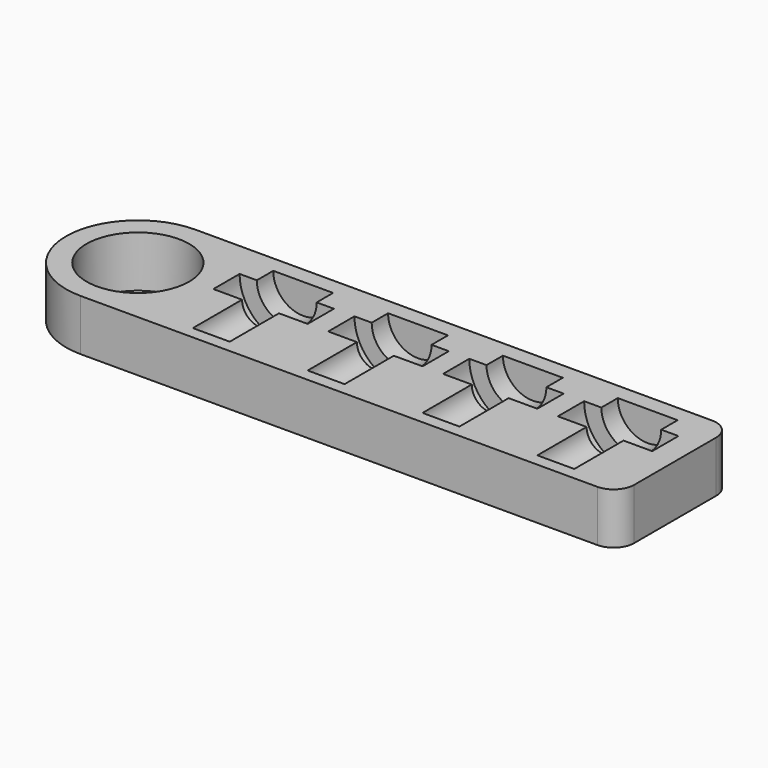
from build123d import *

# Parameters (mm, degrees)
F0_R         = 12.5
F1_DEPTH     = 12.5
F7_TEXT_SIZE = 5.5555555556
F8_DEPTH     = 1


# Not quite as in the source:
# - Text() gives the source's letters only with a copy of the font that has no kerning and outlines rounded to 1/6400 em; it was checked with that copy


with BuildPart() as f1:
    # F0 (on Top) → F1 (new body)
    with BuildSketch(Plane.XY):
        with BuildLine():
            ThreePointArc((0, 17.5), (5.1256313292, 5.1256313292), (17.5, 0))
            Line((17.5, 0), (143.5, 0))
            ThreePointArc((143.5, 0), (147.0355339059, 1.4644660941), (148.5, 5))
            Line((148.5, 5), (148.5, 30))
            ThreePointArc((148.5, 30), (147.0355339059, 33.5355339059), (143.5, 35))
            Line((143.5, 35), (17.5, 35))
            ThreePointArc((17.5, 35), (5.1256313292, 29.8743686708), (0, 17.5))
        make_face()
        with Locations((17.5, 17.5)):
            Circle(F0_R, mode=Mode.SUBTRACT)
    extrude(amount=F1_DEPTH)

    # F2 (on face) → F3 (revolve, cut)
    with BuildSketch(Plane.XY.offset(12.5)):
        Polygon((47, 18), (47, 3), (51.5, 3), (51.5, 18), (58.5, 18), (58.5, 26), (54.3, 26), (54.3, 31), (47, 31), (47, 26), align=None)
    revolve(axis=Axis((47, 10.5, 12.5), (0, 1, 0)), mode=Mode.SUBTRACT)

    # F2 (on face) → F4 (revolve, cut)
    with BuildSketch(Plane.XY.offset(12.5)):
        Polygon((75, 18), (75, 3), (79.5, 3), (79.5, 18), (86.5, 18), (86.5, 26), (82.3, 26), (82.3, 31), (75, 31), (75, 26), align=None)
    revolve(axis=Axis((75, 22, 12.5), (0, 1, 0)), mode=Mode.SUBTRACT)

    # F2 (on face) → F5 (revolve, cut)
    with BuildSketch(Plane.XY.offset(12.5)):
        Polygon((103, 18), (103, 3), (107.5, 3), (107.5, 18), (114.5, 18), (114.5, 26), (110.3, 26), (110.3, 31), (103, 31), (103, 26), align=None)
    revolve(axis=Axis((103, 22, 12.5), (0, 1, 0)), mode=Mode.SUBTRACT)

    # F2 (on face) → F6 (revolve, cut)
    with BuildSketch(Plane.XY.offset(12.5)):
        Polygon((131, 18), (131, 3), (135.5, 3), (135.5, 18), (142.5, 18), (142.5, 26), (138.3, 26), (138.3, 31), (131, 31), (131, 26), align=None)
    revolve(axis=Axis((131, 22, 12.5), (0, 1, 0)), mode=Mode.SUBTRACT)

    # F7 (on face) → F8 (cut)
    with BuildSketch(Plane(origin=(0, 0, 0), x_dir=(1, 0, 0), z_dir=(0, 0, -1))):
        with Locations((30, -9)):
            Text('796', F7_TEXT_SIZE, font='Open Sans', text_align=(TextAlign.LEFT, TextAlign.BOTTOM))
    extrude(amount=-F8_DEPTH, mode=Mode.SUBTRACT)


solid = f1.part
